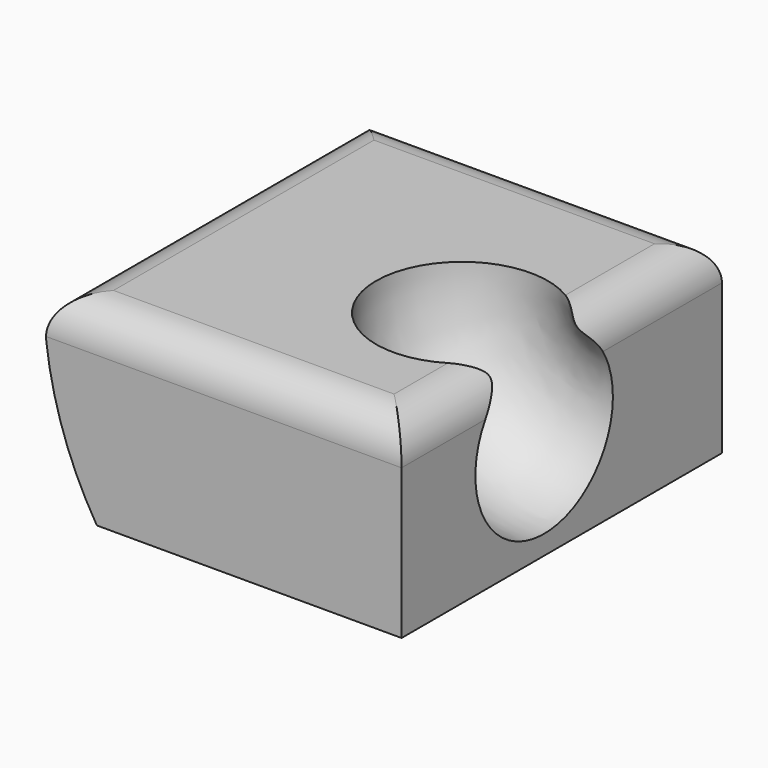
from build123d import *

# Parameters (mm, degrees)
F0_W        = 48.4990663826
F0_H        = 54.2960166931
F1_DEPTH    = 25.4
F4_T1_DEPTH = 73.8990663826
F4_T3_DEPTH = 55.000743558
F4_T5_DEPTH = 60.9725440939
F4_T7_DEPTH = 82.7166388813


# Not quite as in the source:
# - a fillet or chamfer that OpenCascade refuses, or shapes differently, is made with other operations: its cross-section is extruded or revolved along the edge and cut away or added


with BuildPart() as f1:
    # F0 (on Top) → F1 (new body)
    with BuildSketch(Plane.XY):
        with Locations((24.2495331913, 27.1480083466)):
            Rectangle(F0_W, F0_H)
    extrude(amount=F1_DEPTH)

    # F2 (on face) → F3 (revolve, intersect)
    with BuildSketch(Plane.XY.offset(25.4)):
        with BuildLine():
            ThreePointArc((48.4990663826, 20.710743558), (25.7133262446, 24.1621080786), (48.4990663826, 27.6134725992))
            Line((48.4990663826, 27.6134725992), (48.4990663826, 54.2960166931))
            Line((48.4990663826, 54.2960166931), (0, 54.2960166931))
            Line((0, 54.2960166931), (0, 0))
            Line((0, 0), (48.4990663826, 0))
            Line((48.4990663826, 0), (48.4990663826, 20.710743558))
        make_face()
    revolve(axis=Axis((48.4990663826, 27.1480083466, 25.4), (0, 1, 0)), mode=Mode.INTERSECT)

    # F4: fillet of radius 5.08 on 5 edges, made by hand

    # F4_s2 → F4_t1 (cut)
    with BuildSketch(Plane.YZ.offset(-12.7)):
        with BuildLine():
            ThreePointArc((5.08, 25.4), (1.4878975516, 23.9121024484), (0, 20.32))
            Line((0, 20.32), (0, 25.4))
            Line((0, 25.4), (5.08, 25.4))
        make_face()
        with BuildLine():
            ThreePointArc((49.2160166931, 25.4), (52.8081191415, 23.9121024484), (54.2960166931, 20.32))
            Line((54.2960166931, 20.32), (54.2960166931, 25.4))
            Line((54.2960166931, 25.4), (49.2160166931, 25.4))
        make_face()
    extrude(amount=F4_T1_DEPTH, mode=Mode.SUBTRACT)

    # F4_s4 → F4_t3 (cut)
    with BuildSketch(Plane.XZ.offset(-42.300743558)):
        with BuildLine():
            ThreePointArc((43.4190663826, 25.4), (47.0111688311, 23.9121024484), (48.4990663826, 20.32))
            Line((48.4990663826, 20.32), (48.4990663826, 25.4))
            Line((48.4990663826, 25.4), (43.4190663826, 25.4))
        make_face()
    extrude(amount=F4_T3_DEPTH, mode=Mode.SUBTRACT)

    # F4_s6 → F4_t5 (cut)
    with BuildSketch(Plane.XZ.offset(-66.9960166931)):
        with BuildLine():
            ThreePointArc((43.4190663826, 25.4), (47.0111688311, 23.9121024484), (48.4990663826, 20.32))
            Line((48.4990663826, 20.32), (48.4990663826, 25.4))
            Line((48.4990663826, 25.4), (43.4190663826, 25.4))
        make_face()
    extrude(amount=F4_T5_DEPTH, mode=Mode.SUBTRACT)

    # F4_s8 → F4_t7 (cut)
    with BuildSketch(Plane.XZ.offset(-68.5063277872)):
        with BuildLine():
            ThreePointArc((5.3782022269, 25.4), (1.5817742667, 23.6954310455), (0.3330916761, 19.7256435997))
            ThreePointArc((0.3330916761, 19.7256435997), (0.0833445319, 22.5579377812), (0, 25.4))
            Line((0, 25.4), (5.3782022269, 25.4))
        make_face()
    extrude(amount=F4_T7_DEPTH, mode=Mode.SUBTRACT)


solid = f1.part
